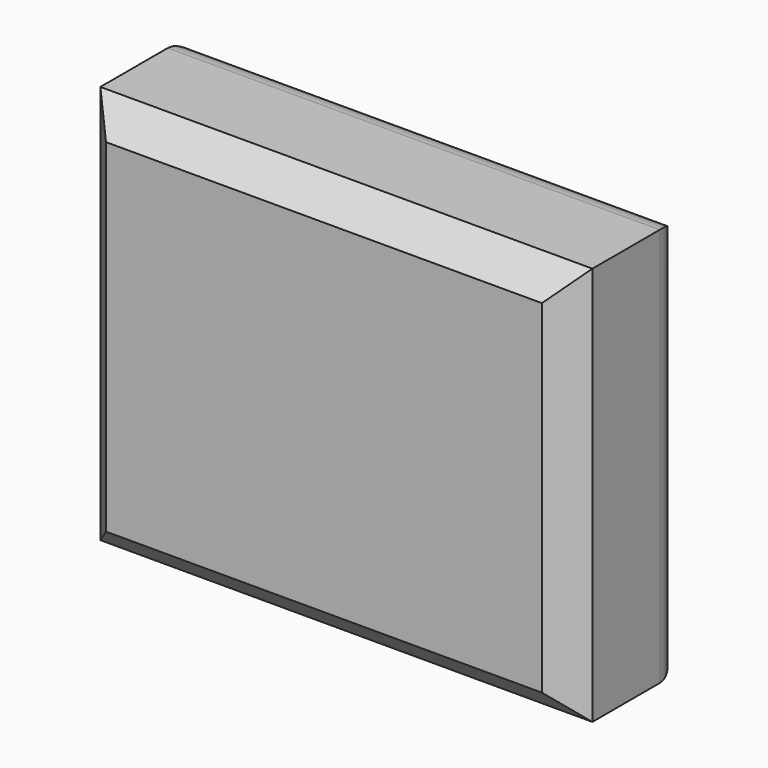
from build123d import *

# Parameters (mm, degrees)
F0_W     = 89.0572415665
F0_H     = 72.2243338823
F1_DEPTH = 25.4
F2_SIZE  = 5.08
F3_R     = 5.08
F4_T     = -2.54


# Not quite as in the source:
# - a shell that OpenCascade refuses in one call is made with other operations: the cavity is built on its own and cut out


with BuildPart() as f1:
    # F0 (on Front) → F1 (new body)
    with BuildSketch(Plane.XZ):
        with Locations((-52.9469675384, -36.1121669412)):
            Rectangle(F0_W, F0_H)
    extrude(amount=F1_DEPTH)

    # F2
    f2_edges = [f1.edges().sort_by_distance(p)[0] for p in [
        (-97.475588, -25.4, -36.112167),
        (-52.946968, -25.4, 0),
        (-8.418347, -25.4, -36.112167),
        (-52.946968, -25.4, -72.224334),
    ]]
    chamfer(f2_edges, length=F2_SIZE)

    # F3
    f3_edges = [f1.edges().sort_by_distance(p)[0] for p in [
        (-8.418347, 0, -36.112167),
        (-52.946968, 0, 0),
        (-97.475588, 0, -36.112167),
        (-52.946968, 0, -72.224334),
    ]]
    fillet(f3_edges, radius=F3_R)

    # F4: a shell. OpenCascade refuses it in one call, so the cavity is built on its own and cut out:
    # the body offset inwards by the wall thickness, plus a prism from it out through each open face.
    f4_core = offset(f1.part, amount=F4_T, mode=Mode.PRIVATE)
    f4_exits = [f4_core.faces().sort_by_distance(p)[0] for p in [
        (-52.946968, -2.54, -36.112167),
    ]]
    add(f4_core, mode=Mode.SUBTRACT)
    extrude(f4_exits, amount=-F4_T, mode=Mode.SUBTRACT)


solid = f1.part
